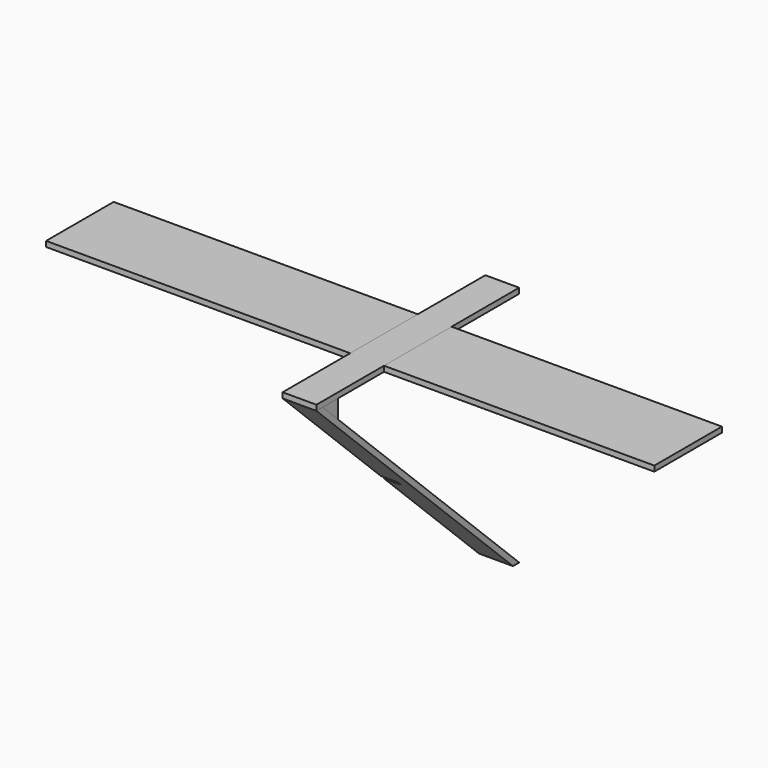
from build123d import *

# Parameters (mm, degrees)
F0_W     = 1800
F0_H     = 250
F1_DEPTH = 16
F3_DEPTH = 100
F4_W     = 50
F4_H     = 16
F5_DEPTH = 16
F6_DEPTH = 100
F8_DEPTH = 16


# Not quite as in the source:
# - the program builds the solid bodies; features that only make, move or delete a surface that nothing else refers to are left out


with BuildPart() as f1:
    # F0 (on Top) → F1 (new body)
    with BuildSketch(Plane.XY):
        Rectangle(F0_W, F0_H)
    extrude(amount=F1_DEPTH)


with BuildPart() as f3:
    # F2 (on Right) → F3 (new body)
    with BuildSketch(Plane.YZ):
        Polygon((-351.933169445, 0), (-375, 0), (351.933169445, -700), (375, -700), align=None)
    extrude(amount=F3_DEPTH)

    # F4 (on face) → F5 (cut, through all)
    with BuildSketch(Plane(origin=(0, -169.3262597137, -175.8412494914), x_dir=(1, 0, 0), z_dir=(0, 0.6936366902, 0.7203250252))):
        with Locations((25, 242.772841577)):
            Rectangle(F4_W, F4_H)
    extrude(amount=-F5_DEPTH, mode=Mode.SUBTRACT)


with BuildPart() as f6:
    # F2 (on Right) → F6 (new body, through all)
    with BuildSketch(Plane.YZ):
        Polygon((-375, 16), (-375, 0), (-351.933169445, 0), (375, 0), (375, 16), align=None)
    extrude(amount=F6_DEPTH)


with BuildPart() as f8:
    # F7 (on face) → F8 (new body)
    with BuildSketch(Plane.YZ.offset(100)):
        Polygon((-294.8169918458, 0), (-351.933169445, 0), (-294.8169918458, -55), align=None)
    extrude(amount=-F8_DEPTH)


solid = Compound([f1.part, f3.part, f6.part, f8.part])
